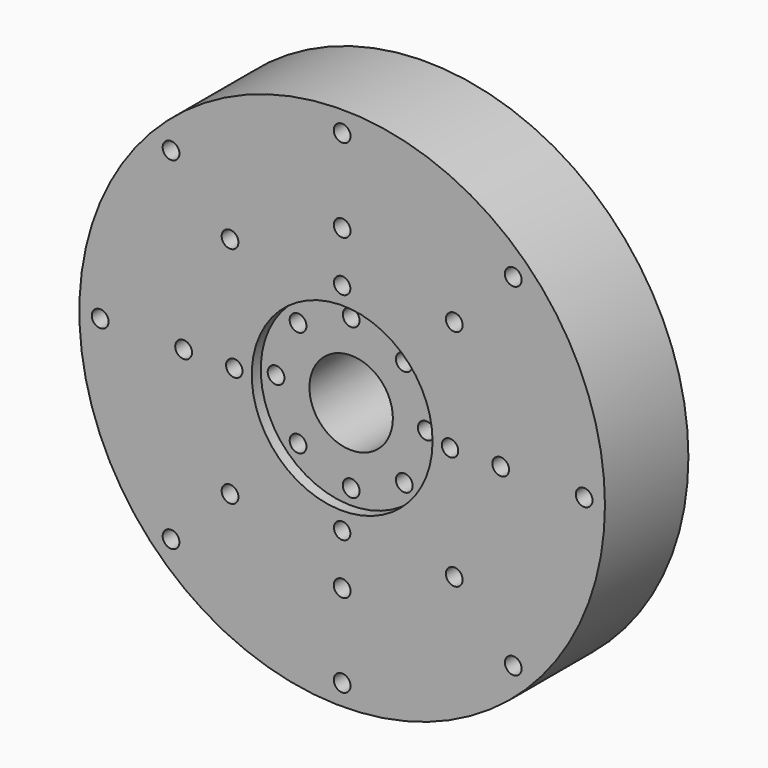
from build123d import *

# Parameters (mm, degrees)
F0_R     = 80
F0_R_2   = 2.5527
F0_R_3   = 39.9796
F0_R_4   = 2.5
F0_R_5   = 27.5209
F0_R_6   = 12.7
F1_DEPTH = 31.75
F2_DEPTH = 12.7
F3_DEPTH = 3.429


# Not quite as in the source:
# - a feature names something its author has since deleted; it is built from what else it names


with BuildPart() as f1:
    # F0 (on Front) → F1 (new body)
    with BuildSketch(Plane.XZ):
        Circle(F0_R)
        with Locations((-52.0854855022, -52.0854855022)):
            Circle(F0_R_2, mode=Mode.SUBTRACT)
        with Locations((-34.1249732601, -34.1249732601)):
            Circle(F0_R_2, mode=Mode.SUBTRACT)
        with Locations((0, -73.66)):
            Circle(F0_R_2, mode=Mode.SUBTRACT)
        with Locations((0, -48.26)):
            Circle(F0_R_2, mode=Mode.SUBTRACT)
        with Locations((52.0854855022, -52.0854855022)):
            Circle(F0_R_2, mode=Mode.SUBTRACT)
        with Locations((34.1249732601, -34.1249732601)):
            Circle(F0_R_2, mode=Mode.SUBTRACT)
        with Locations((-73.66, 0)):
            Circle(F0_R_2, mode=Mode.SUBTRACT)
        with Locations((-48.26, 0)):
            Circle(F0_R_2, mode=Mode.SUBTRACT)
        with Locations((-34.1249732601, 34.1249732601)):
            Circle(F0_R_2, mode=Mode.SUBTRACT)
        with Locations((-52.0854855022, 52.0854855022)):
            Circle(F0_R_2, mode=Mode.SUBTRACT)
        Circle(F0_R_3, mode=Mode.SUBTRACT)
        with Locations((34.1249732601, 34.1249732601)):
            Circle(F0_R_2, mode=Mode.SUBTRACT)
        with Locations((48.26, 0)):
            Circle(F0_R_2, mode=Mode.SUBTRACT)
        with Locations((73.66, 0)):
            Circle(F0_R_2, mode=Mode.SUBTRACT)
        with Locations((0, 48.26)):
            Circle(F0_R_2, mode=Mode.SUBTRACT)
        with Locations((0, 73.66)):
            Circle(F0_R_2, mode=Mode.SUBTRACT)
        with Locations((52.0854855022, 52.0854855022)):
            Circle(F0_R_2, mode=Mode.SUBTRACT)
        Circle(F0_R_3)
        with Locations((0, -32.8422)):
            Circle(F0_R_4, mode=Mode.SUBTRACT)
        with Locations((-32.8422, 0)):
            Circle(F0_R_4, mode=Mode.SUBTRACT)
        Circle(F0_R_5, mode=Mode.SUBTRACT)
        with Locations((32.8422, 0)):
            Circle(F0_R_4, mode=Mode.SUBTRACT)
        with Locations((0, 32.8422)):
            Circle(F0_R_4, mode=Mode.SUBTRACT)
        Circle(F0_R_5)
        with Locations((-16.1644610179, -16.1644610179)):
            Circle(F0_R_2, mode=Mode.SUBTRACT)
        with Locations((0, -22.86)):
            Circle(F0_R_2, mode=Mode.SUBTRACT)
        with Locations((16.1644610179, -16.1644610179)):
            Circle(F0_R_2, mode=Mode.SUBTRACT)
        with Locations((-22.86, 0)):
            Circle(F0_R_2, mode=Mode.SUBTRACT)
        with Locations((-16.1644610179, 16.1644610179)):
            Circle(F0_R_2, mode=Mode.SUBTRACT)
        Circle(F0_R_6, mode=Mode.SUBTRACT)
        with Locations((16.1644610179, 16.1644610179)):
            Circle(F0_R_2, mode=Mode.SUBTRACT)
        with Locations((22.86, 0)):
            Circle(F0_R_2, mode=Mode.SUBTRACT)
        with Locations((0, 22.86)):
            Circle(F0_R_2, mode=Mode.SUBTRACT)
        with Locations((0, 32.8422)):
            Circle(F0_R_4)
        with Locations((0, -32.8422)):
            Circle(F0_R_4)
        with Locations((32.8422, 0)):
            Circle(F0_R_4)
        with Locations((-32.8422, 0)):
            Circle(F0_R_4)
    extrude(amount=-F1_DEPTH)

    # F0 (on Front) → F2 (cut)
    with BuildSketch(Plane.XZ):
        with Locations((0, 32.8422)):
            Circle(F0_R_4)
        with Locations((32.8422, 0)):
            Circle(F0_R_4)
        with Locations((0, -32.8422)):
            Circle(F0_R_4)
        with Locations((-32.8422, 0)):
            Circle(F0_R_4)
    extrude(amount=-F2_DEPTH, mode=Mode.SUBTRACT)

    # F0 (on Front) → F3 (cut)
    with BuildSketch(Plane.XZ):
        Circle(F0_R_5)
        with Locations((-16.1644610179, -16.1644610179)):
            Circle(F0_R_2, mode=Mode.SUBTRACT)
        with Locations((0, -22.86)):
            Circle(F0_R_2, mode=Mode.SUBTRACT)
        with Locations((16.1644610179, -16.1644610179)):
            Circle(F0_R_2, mode=Mode.SUBTRACT)
        with Locations((-22.86, 0)):
            Circle(F0_R_2, mode=Mode.SUBTRACT)
        with Locations((-16.1644610179, 16.1644610179)):
            Circle(F0_R_2, mode=Mode.SUBTRACT)
        Circle(F0_R_6, mode=Mode.SUBTRACT)
        with Locations((16.1644610179, 16.1644610179)):
            Circle(F0_R_2, mode=Mode.SUBTRACT)
        with Locations((22.86, 0)):
            Circle(F0_R_2, mode=Mode.SUBTRACT)
        with Locations((0, 22.86)):
            Circle(F0_R_2, mode=Mode.SUBTRACT)
    extrude(amount=-F3_DEPTH, mode=Mode.SUBTRACT)


solid = f1.part
